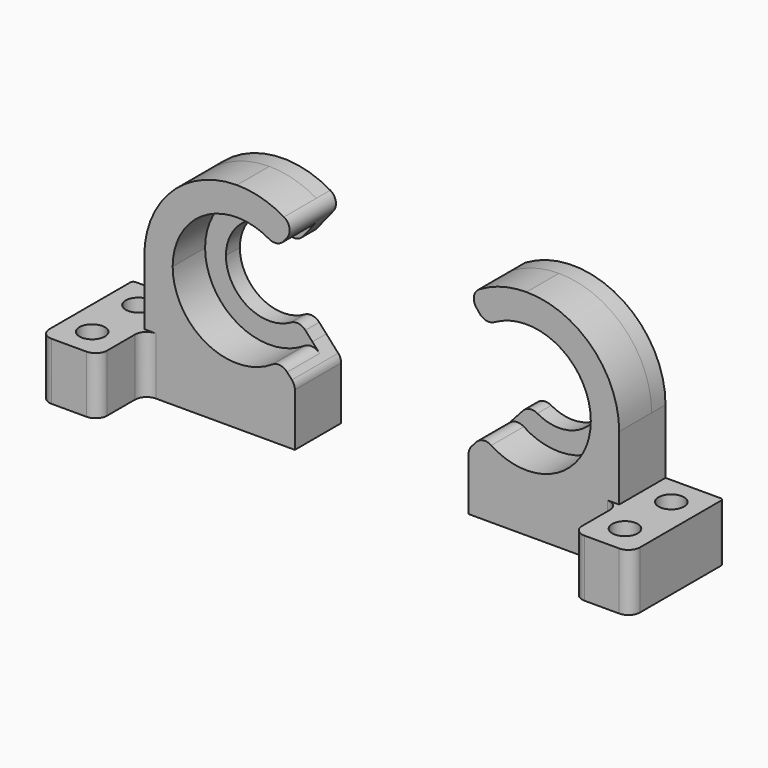
from build123d import *

# Parameters (mm, degrees)
F1_DEPTH = 7
F2_DEPTH = 3
F3_W     = 10
F3_H     = 9.9
F4_DEPTH = 10
F6_D     = 4.4
F7_R     = 2
F8_R     = 2
F9_R     = 0.5


# Not quite as in the source:
# - a feature names something its author has since deleted; it is built from what else it names


with BuildPart() as f1:
    # F0 (on Front) → F1 (new body)
    with BuildSketch(Plane.XZ):
        with BuildLine():
            ThreePointArc((-10, -12.4899959968), (1.031140389, -15.9667388498), (11.5234543432, -11.1))
            Line((11.5234543432, -11.1), (0, -11.1))
            Line((0, -11.1), (-10, -11.1))
            Line((-10, -11.1), (-10, -12.4899959968))
        make_face()
        with BuildLine():
            Line((26, -21), (26, -11.1))
            Line((26, -11.1), (16, -11.1))
            Line((16, -11.1), (11.5234543432, -11.1))
            ThreePointArc((11.5234543432, -11.1), (1.031140389, -15.9667388498), (-10, -12.4899959968))
            Line((-10, -12.4899959968), (-10, -21))
            Line((-10, -21), (26, -21))
        make_face()
        with BuildLine():
            Line((16, -11.1), (16, 0))
            ThreePointArc((16, 0), (14.8387207921, -5.9843433436), (11.5234543432, -11.1))
            Line((11.5234543432, -11.1), (16, -11.1))
        make_face()
        with BuildLine():
            ThreePointArc((16, 0), (11.313708499, 11.313708499), (0, 16))
            ThreePointArc((0, 16), (-5.2990595416, 15.0970185128), (-10, 12.4899959968))
            Line((-10, 12.4899959968), (-6.9375, 8.6649347228))
            ThreePointArc((-6.9375, 8.6649347228), (4.806440991, 10.0054047894), (11.1, 0))
            ThreePointArc((11.1, 0), (7.8488852712, -7.8488852712), (0, -11.1))
            Line((0, -11.1), (11.5234543432, -11.1))
            ThreePointArc((11.5234543432, -11.1), (14.8387207921, -5.9843433436), (16, 0))
        make_face()
        with BuildLine():
            Line((-7.4296123602, -8.2468697199), (-10, -11.1))
            Line((-10, -11.1), (0, -11.1))
            ThreePointArc((0, -11.1), (-3.9793055996, -10.3621970134), (-7.4296123602, -8.2468697199))
        make_face()
    extrude(amount=F1_DEPTH)

    # F1_face (on face) + F0 (on Front) → F2 (join)
    with BuildSketch(Plane(origin=(7.471830613, 0, -8.1748565064), x_dir=(1, 0, 0), z_dir=(0, 1, 0))):
        with BuildLine():
            Line((-17.471830613, 2.9251434936), (-14.9014429732, 0.0720132135))
            ThreePointArc((-14.9014429732, 0.0720132135), (3.6234729777, -7.8519970471), (-14.409330613, -16.8397912292))
            Line((-14.409330613, -16.8397912292), (-17.471830613, -20.6648525032))
            ThreePointArc((-17.471830613, -20.6648525032), (-0.5436273827, -22.5970616082), (8.528169387, -8.1748565064))
            Line((8.528169387, -8.1748565064), (8.528169387, 2.9251434936))
            Line((8.528169387, 2.9251434936), (18.528169387, 2.9251434936))
            Line((18.528169387, 2.9251434936), (18.528169387, 12.8251434936))
            Line((18.528169387, 12.8251434936), (-17.471830613, 12.8251434936))
            Line((-17.471830613, 12.8251434936), (-17.471830613, 2.9251434936))
        make_face()
    with BuildSketch(Plane.XZ):
        with BuildLine():
            ThreePointArc((11.1, 0), (4.806440991, 10.0054047894), (-6.9375, 8.6649347228))
            Line((-6.9375, 8.6649347228), (-4.6875, 5.8546856235))
            ThreePointArc((-4.6875, 5.8546856235), (3.2475952642, 6.7604086415), (7.5, 0))
            ThreePointArc((7.5, 0), (3.0495850016, -6.8520092906), (-5.0200083515, -5.5722092702))
            Line((-5.0200083515, -5.5722092702), (-7.4296123602, -8.2468697199))
            ThreePointArc((-7.4296123602, -8.2468697199), (-3.9793055996, -10.3621970134), (0, -11.1))
            ThreePointArc((0, -11.1), (7.8488852712, -7.8488852712), (11.1, 0))
        make_face()
    extrude(amount=F2_DEPTH, dir=(0, 1, 0))

    # F3 (on face) → F4 (join)
    with BuildSketch(Plane.XZ.offset(7)):
        with Locations((21, -16.05)):
            Rectangle(F3_W, F3_H)
    extrude(amount=F4_DEPTH)

    # F6 (through all)
    with Locations(Plane.XY.offset(-11.1)):
        with Locations((21, -2), (21, -12)):
            Hole(F6_D / 2)

    # F7
    f7_edges = [f1.edges().sort_by_distance(p)[0] for p in [
        (-10, -2, 12.489996),
        (-4.6875, 1.5, 5.854686),
        (-5.020008, 1.5, -5.572209),
        (-7.429612, -3.5, -8.24687),
        (-6.9375, -3.5, 8.664935),
        (-10, -2, -11.1),
    ]]
    fillet(f7_edges, radius=F7_R)

    # F8
    f8_edges = [f1.edges().sort_by_distance(p)[0] for p in [
        (16, -17, -16.05),
        (16, -7, -16.05),
        (26, -17, -16.05),
    ]]
    fillet(f8_edges, radius=F8_R)

    # F9
    f9_edges = [f1.edges().sort_by_distance(p)[0] for p in [
        (26, 3, -16.05),
    ]]
    fillet(f9_edges, radius=F9_R)


with BuildPart() as f11_1:
    # F11: instance of F1
    add(f1.part.mirror(Plane.YZ.offset(-25)))


solid = Compound([f1.part, f11_1.part])
